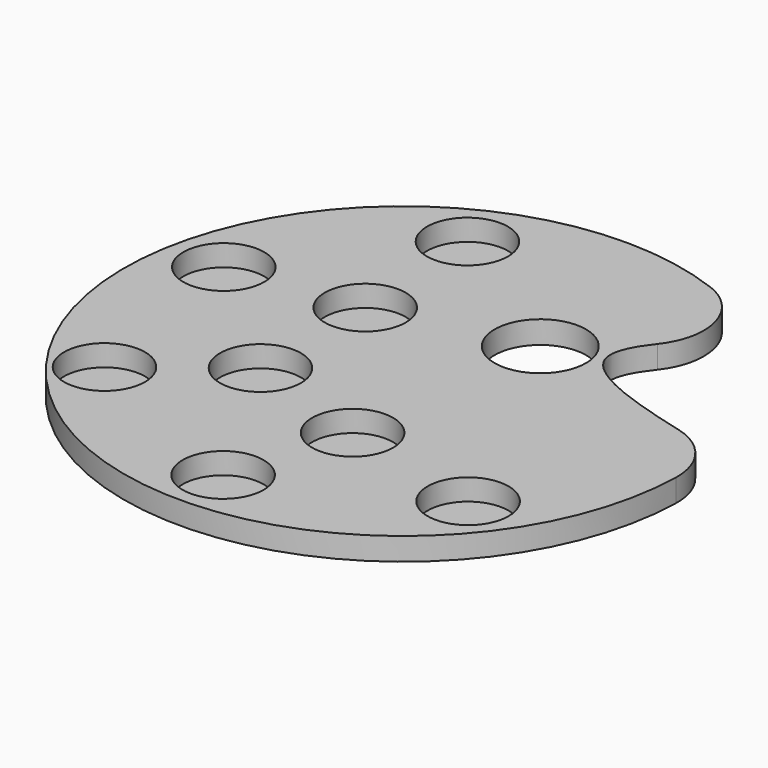
from build123d import *

# Parameters (mm, degrees)
F1_DEPTH = 3.5
F2_R     = 7.058260031
F3_DEPTH = 25
F4_R     = 6.25
F5_DEPTH = 3.3
F6_R     = 6.25
F7_DEPTH = 3.3
F8_R     = 10


with BuildPart() as f1:
    # F0 (on Top) → F1 (new body)
    with BuildSketch(Plane.XY):
        with BuildLine():
            add(Edge.make_bspline(
                [(27.7347816335, 32.9664582942), (21.7968576271, 27.4921287364), (8.5785934713, 15.3075413902), (30.4614719911, 10.0037248917), (42.4955969964, 7.0802345045)],
                knots=[0, 0, 0, 0, 0.4495258402, 1, 1, 1, 1], degree=3))
            ThreePointArc((27.7347816335, 32.9664582942), (-37.424599746, -21.3402159917), (42.4955969964, 7.0802345045))
        make_face()
    extrude(amount=F1_DEPTH)

    # F2 (on Top) → F3 (cut)
    with BuildSketch(Plane.XY):
        with Locations((8.8732391596, 15.4273370281)):
            Circle(F2_R)
    extrude(amount=F3_DEPTH, mode=Mode.SUBTRACT)

    # F4 (on face) → F5 (cut)
    with BuildSketch(Plane.XY.offset(3.5)):
        with Locations((-15.0699157128, 31.2930024222)):
            Circle(F4_R)
        with Locations((-33.8617932364, 7.7287333374)):
            Circle(F4_R)
        with Locations((-28.7774891506, -21.6554295879)):
            Circle(F4_R)
        with Locations((0, -34.7326123432)):
            Circle(F4_R)
        with Locations((27.3688023133, -21.6334286339)):
            Circle(F4_R)
    extrude(amount=-F5_DEPTH, mode=Mode.SUBTRACT)

    # F6 (on face) → F7 (cut)
    with BuildSketch(Plane.XY.offset(3.5)):
        with Locations((-13.9189545551, -10.1127124297)):
            Circle(F6_R)
        with Locations((5.3165675522, -16.3627124297)):
            Circle(F6_R)
        with Locations((-13.9189545551, 10.1127124297)):
            Circle(F6_R)
    extrude(amount=-F7_DEPTH, mode=Mode.SUBTRACT)

    # F8
    f8_edges = [f1.edges().sort_by_distance(p)[0] for p in [
        (27.734782, 32.966458, 1.75),
        (42.495597, 7.080235, 1.75),
    ]]
    fillet(f8_edges, radius=F8_R)


solid = f1.part
